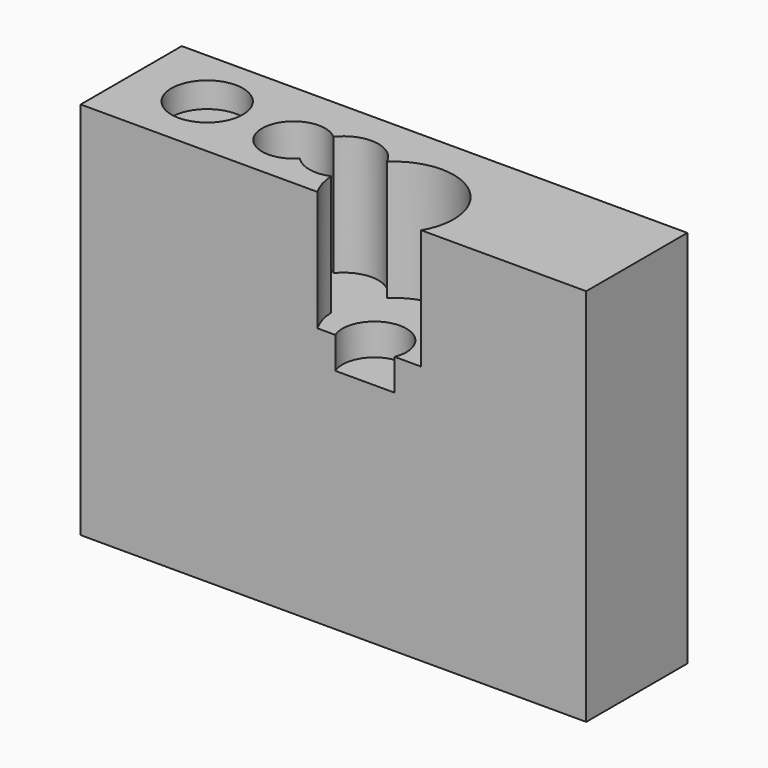
from build123d import *

# Parameters (mm, degrees)
F0_W      = 2000
F0_H      = 500
F1_DEPTH  = 1500
F2_R      = 141.1964442428
F3_DEPTH  = 100
F4_R      = 34.4012155817
F1_FACE_W = 2000
F1_FACE_H = 500
F1_FACE_R = 141.1964442428
F5_DEPTH  = 300
F6_R      = 22.2612942047
F7_DEPTH  = 25
F11_DEPTH = 25
F12_DEPTH = 500
F13_R     = 126.398375951
F14_DEPTH = 600


# Not quite as in the source:
# - a feature of the source that left no trace in its solid (it failed there, or was rolled back) is left out


with BuildPart() as f1:
    # F0 (on Top) → F1 (new body)
    with BuildSketch(Plane.XY):
        with Locations((-90.5123054981, -534.5377490795)):
            Rectangle(F0_W, F0_H)
    extrude(amount=-F1_DEPTH)

    # F2 (on Top) → F3 (cut)
    with BuildSketch(Plane.XY):
        with Locations((-797.8549599648, -524.8737335205)):
            Circle(F2_R)
    extrude(amount=-F3_DEPTH, mode=Mode.SUBTRACT)

    # F4 (on face) + F1_face (on face) → F5 (cut)
    with BuildSketch(Plane.XY.offset(-100)):
        with Locations((-826.4881968498, -472.618997097)):
            Circle(F4_R)
    with BuildSketch(Plane(origin=(-43.2497509657, -535.1834701589, 0), x_dir=(1, 0, 0), z_dir=(0, 0, 1))):
        with Locations((-47.2625545324, 0.6457210794)):
            Rectangle(F1_FACE_W, F1_FACE_H)
        with Locations((-754.605208999, 10.3097366384)):
            Circle(F1_FACE_R, mode=Mode.SUBTRACT)
    extrude(amount=F5_DEPTH, mode=Mode.SUBTRACT)

    # F6 (on Top) → F7 (cut)
    with BuildSketch(Plane.XY):
        with Locations((-837.3667597771, -527.3413062096)):
            Circle(F6_R)
    extrude(amount=-F7_DEPTH, mode=Mode.SUBTRACT)

    # F10 (on Top) → F11 (join)
    with BuildSketch(Plane.XY):
        with BuildLine():
            ThreePointArc((-336.3280592399, -643.7038848361), (-311.8886426753, -604.522487328), (-303.3533888527, -559.1394901276))
            ThreePointArc((-303.3533888527, -559.1394901276), (-314.3656518823, -507.8553931627), (-345.4608968402, -465.6130651073))
            ThreePointArc((-345.4608968402, -465.6130651073), (-373.9207280875, -556.3521241934), (-336.3280592399, -643.7038848361))
        make_face()
        with BuildLine():
            ThreePointArc((-345.4608968402, -465.6130651073), (-314.3656518823, -507.8553931627), (-303.3533888527, -559.1394901276))
            ThreePointArc((-303.3533888527, -559.1394901276), (-311.8886426753, -604.522487328), (-336.3280592399, -643.7038848361))
            ThreePointArc((-336.3280592399, -643.7038848361), (-266.2138077643, -683.0061743425), (-186.1307836251, -676.1223189436))
            ThreePointArc((-186.1307836251, -676.1223189436), (-169.5365195374, -576.3659050684), (-113.0004686355, -492.5185040457))
            ThreePointArc((-113.0004686355, -492.5185040457), (-221.6444367274, -413.5213420531), (-345.4608968402, -465.6130651073))
        make_face()
        with BuildLine():
            ThreePointArc((-336.3280592399, -643.7038848361), (-373.9207280875, -556.3521241934), (-345.4608968402, -465.6130651073))
            ThreePointArc((-345.4608968402, -465.6130651073), (-553.0316980704, -565.5372770485), (-336.3280592399, -643.7038848361))
        make_face()
        with BuildLine():
            ThreePointArc((289.3120863194, -664.3842458725), (144.8913865697, -445.641688806), (-113.0004686355, -492.5185040457))
            ThreePointArc((-113.0004686355, -492.5185040457), (-103.7589334647, -520.2685961551), (-100.6307099798, -549.3493080139))
            ThreePointArc((-100.6307099798, -549.3493080139), (-124.0033138355, -625.8046199509), (-186.1307836251, -676.1223189436))
            ThreePointArc((-186.1307836251, -676.1223189436), (57.3165773299, -902.1781192905), (289.3120863194, -664.3842458725))
        make_face()
        with BuildLine():
            ThreePointArc((-100.6307099798, -549.3493080139), (-103.7589334647, -520.2685961551), (-113.0004686355, -492.5185040457))
            ThreePointArc((-113.0004686355, -492.5185040457), (-169.5365195374, -576.3659050684), (-186.1307836251, -676.1223189436))
            ThreePointArc((-186.1307836251, -676.1223189436), (-124.0033138355, -625.8046199509), (-100.6307099798, -549.3493080139))
        make_face()
    extrude(amount=F11_DEPTH)

    # F12 (cut): a face of the model
    f12_faces = [f1.faces().sort_by_distance(p)[0] for p in [
        (-80.6836957397, -625.9699801923, 25),
    ]]
    extrude(f12_faces, amount=-F12_DEPTH, mode=Mode.SUBTRACT)

    # F13 (on Top) → F14 (cut)
    with BuildSketch(Plane.XY):
        with Locations((34.1630466282, -737.5611066818)):
            Circle(F13_R)
    extrude(amount=-F14_DEPTH, mode=Mode.SUBTRACT)


solid = f1.part
